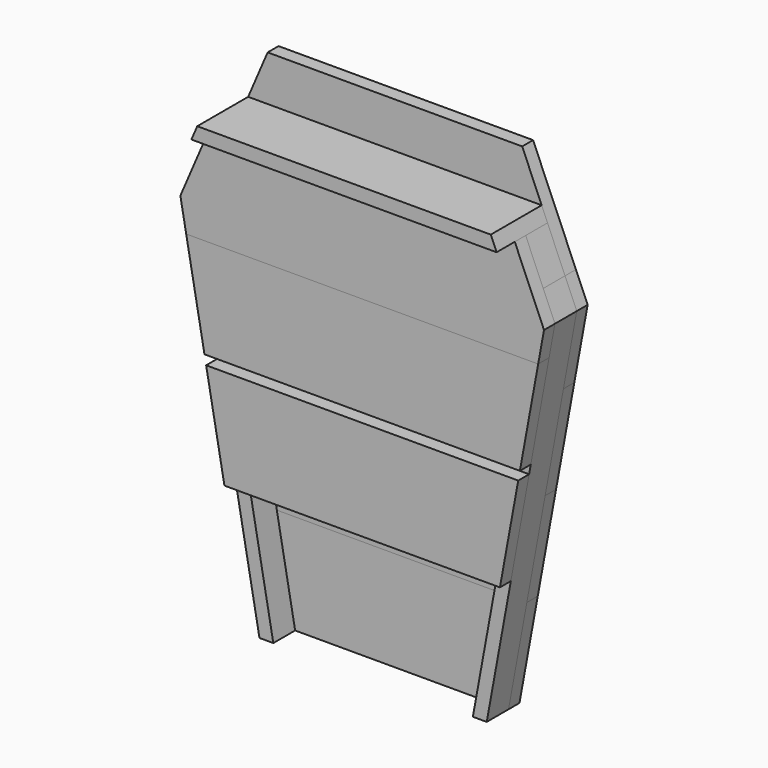
from build123d import *

# Parameters (mm, degrees)
F2_DEPTH  = 19.05
F3_DEPTH  = 19.05
F5_DEPTH  = 38.1
F6_DEPTH  = 38.1
F7_DEPTH  = 88.9
F9_DEPTH  = 19.05
F10_DEPTH = 19.05


# Not quite as in the source:
# - a feature names something its author has since deleted; it is built from what else it names


with BuildPart() as f2:
    # F1 (on Front) → F2 (new body)
    with BuildSketch(Plane.XZ):
        Polygon((-209.8597560976, -419.1), (-184.3048780488, -558.8), (184.3048780488, -558.8), (209.8597560976, -419.1), align=None)
    extrude(amount=F2_DEPTH)


with BuildPart() as f2b:
    # F1 (on Front) → F2, piece 2 (new body)
    with BuildSketch(Plane.XZ):
        Polygon((-254, -177.8), (-235.4146341463, -279.4), (235.4146341463, -279.4), (254, -177.8), (237.6714285714, -139.7), (-237.6714285714, -139.7), align=None)
    extrude(amount=F2_DEPTH)


with BuildPart() as f3:
    # F1 (on Front) → F3 (new body)
    with BuildSketch(Plane.XZ):
        Polygon((-184.3048780488, -558.8), (-158.75, -698.5), (158.75, -698.5), (184.3048780488, -558.8), align=None)
    extrude(amount=F3_DEPTH)


with BuildPart() as f3b:
    # F1 (on Front) → F3, piece 2 (new body)
    with BuildSketch(Plane.XZ):
        Polygon((-235.4146341463, -279.4), (-209.8597560976, -419.1), (209.8597560976, -419.1), (235.4146341463, -279.4), align=None)
    extrude(amount=F3_DEPTH)


with BuildPart() as f3c:
    # F1 (on Front) → F3, piece 3 (new body)
    with BuildSketch(Plane.XZ):
        Polygon((-177.8, 0), (-237.6714285714, -139.7), (237.6714285714, -139.7), (177.8, 0), align=None)
    extrude(amount=F3_DEPTH)


with BuildPart() as f5:
    # F4 (on face) → F5 (new body)
    with BuildSketch(Plane.XZ.offset(19.05)):
        Polygon((-213.1785714286, -82.55), (-237.6714285714, -139.7), (-216.9456460476, -139.7), (-192.4527889048, -82.55), align=None)
        Polygon((-237.6714285714, -139.7), (-254, -177.8), (-234.2271538208, -180.0235181374), (-216.9456460476, -139.7), align=None)
    extrude(amount=F5_DEPTH)


with BuildPart() as f5b:
    # F4 (on face) → F5, piece 2 (new body)
    with BuildSketch(Plane.XZ.offset(19.05)):
        Polygon((192.4527889048, -82.55), (216.9456460476, -139.7), (237.6714285714, -139.7), (213.1785714286, -82.55), align=None)
        Polygon((237.6714285714, -139.7), (216.9456460476, -139.7), (234.2271538208, -180.0235181374), (254, -177.8), align=None)
    extrude(amount=F5_DEPTH)


with BuildPart() as f6:
    # F4 (on face) → F6 (new body)
    with BuildSketch(Plane.XZ.offset(19.05)):
        Polygon((-254, -177.8), (-158.75, -698.5), (-139.3838949435, -698.5), (-234.2271538208, -180.0235181374), align=None)
    extrude(amount=F6_DEPTH)


with BuildPart() as f6b:
    # F4 (on face) → F6, piece 2 (new body)
    with BuildSketch(Plane.XZ.offset(19.05)):
        Polygon((254, -177.8), (234.2271538208, -180.0235181374), (139.3838949435, -698.5), (158.75, -698.5), align=None)
    extrude(amount=F6_DEPTH)


with BuildPart() as f7:
    # F4 (on face) → F7 (new body)
    with BuildSketch(Plane.XZ.offset(19.05)):
        Polygon((-205.0142857143, -63.5), (-213.1785714286, -82.55), (-192.4527889048, -82.55), (192.4527889048, -82.55), (213.1785714286, -82.55), (205.0142857143, -63.5), align=None)
    extrude(amount=F7_DEPTH)


with BuildPart() as f9:
    # F8 (on face) → F9 (new body)
    with BuildSketch(Plane.XZ.offset(57.15)):
        Polygon((192.4527889048, -82.55), (-213.1785714286, -82.55), (-254, -177.8), (-245.868902439, -222.25), (245.868902439, -222.25), (254, -177.8), (234.2271538208, -180.0235181374), align=None)
        Polygon((213.1785714286, -82.55), (192.4527889048, -82.55), (234.2271538208, -180.0235181374), (254, -177.8), align=None)
    extrude(amount=F9_DEPTH)


with BuildPart() as f9b:
    # F8 (on face) → F9, piece 2 (new body)
    with BuildSketch(Plane.XZ.offset(57.15)):
        Polygon((217.9908536585, -374.65), (-217.9908536585, -374.65), (-192.4359756098, -514.35), (192.4359756098, -514.35), align=None)
    extrude(amount=F9_DEPTH)


with BuildPart() as f10:
    # F8 (on face) → F10 (new body)
    with BuildSketch(Plane.XZ.offset(57.15)):
        Polygon((245.868902439, -222.25), (-245.868902439, -222.25), (-220.3140243902, -361.95), (220.3140243902, -361.95), align=None)
    extrude(amount=F10_DEPTH)


solid = Compound([f2.part, f2b.part, f3.part, f3b.part, f3c.part, f5.part, f5b.part, f6.part, f6b.part, f7.part, f9.part, f9b.part, f10.part])
